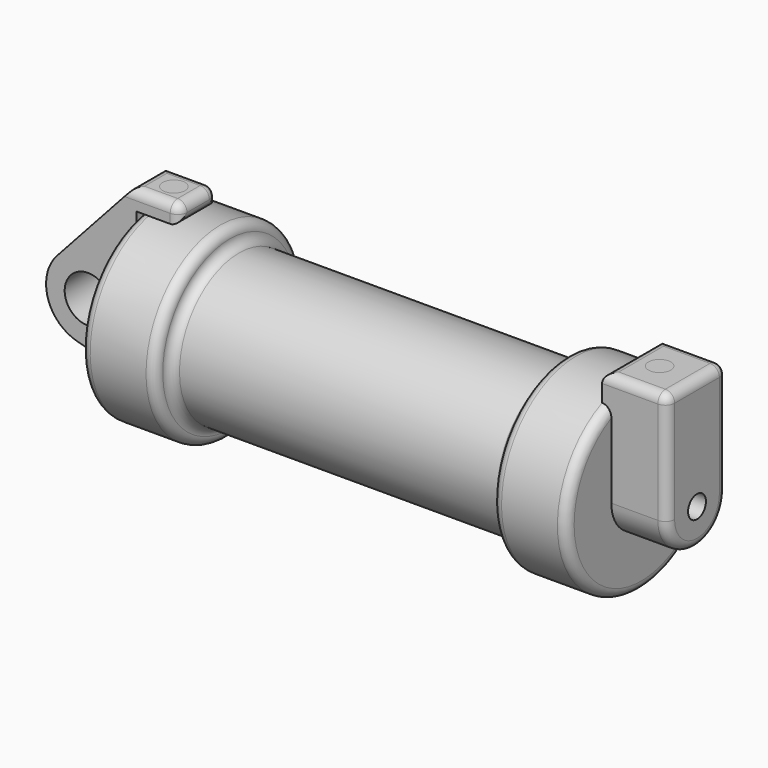
from build123d import *

# Parameters (mm, degrees)
F0_W          = 5.842
F0_H          = 12.7
F0_R          = 3.175
F2_DEPTH      = 3.175
F3_R          = 1.524
F4_DEPTH      = 7.62
F4_DEPTH_BACK = 1.27
F5_R          = 1.524
F6_DEPTH      = 17.78
F7_R          = 1.524
F8_DEPTH      = 10.414
F9_R          = 1.26999
F9_2_R        = 1.26999


# Not quite as in the source:
# - a fillet or chamfer is up to 0.001 mm smaller than in the source, because OpenCascade refuses the exact size


with BuildPart() as f1:
    # F0 (on Front) → F1 (revolve)
    with BuildSketch(Plane.XZ):
        Polygon((5.842, 12.7), (5.842, 0), (66.294, 0), (66.294, 12.7), (56.134, 12.7), (56.134, 10.16), (10.16, 10.16), (10.16, 12.7), align=None)
        with Locations((2.921, 6.35)):
            Rectangle(F0_W, F0_H)
    revolve(axis=Axis((33.147, 0, 0), (-1, 0, 0)))

    # F3 (on face) → F4 (join, two sides)
    with BuildSketch(Plane.YZ.offset(66.294)) as f4_sk:
        with BuildLine():
            ThreePointArc((-5.08, 0), (0, 5.08), (5.08, 0))
            Line((5.08, 0), (5.08, 11.6397422652))
            ThreePointArc((5.08, 11.6397422652), (0, 12.7), (-5.08, 11.6397422652))
            Line((-5.08, 11.6397422652), (-5.08, 0))
        make_face()
        with BuildLine():
            ThreePointArc((-5.08, 0), (0, -5.08), (5.08, 0))
            ThreePointArc((5.08, 0), (0, 5.08), (-5.08, 0))
        make_face()
        Circle(F3_R, mode=Mode.SUBTRACT)
        with BuildLine():
            ThreePointArc((-5.08, 11.6397422652), (0, 12.7), (5.08, 11.6397422652))
            Line((5.08, 11.6397422652), (5.08, 15.24))
            Line((5.08, 15.24), (-5.08, 15.24))
            Line((-5.08, 15.24), (-5.08, 11.6397422652))
        make_face()
    extrude(amount=F4_DEPTH)
    extrude(f4_sk.sketch, amount=-F4_DEPTH_BACK)

    # F9 (radius 1.27 in the source; OpenCascade refuses exactly that, so slightly less here)
    f9_edges = [f1.edges().sort_by_distance(p)[0] for p in [
        (10.16, 0, -12.7),
        (0, 0, -12.7),
        (10.16, 0, -10.16),
        (56.134, 0, -10.16),
        (33.147, 0, 10.16),
        (73.914, 0, 15.24),
        (69.469, 5.08, 15.24),
        (65.024, 0, 15.24),
        (69.469, -5.08, 15.24),
        (56.134, 0, -12.7),
        (66.294, 0, -12.7),
        (73.914, -5.08, 7.62),
        (73.914, 5.08, 7.62),
        (73.914, 0, -5.08),
    ]]
    fillet(f9_edges, radius=F9_R)


with BuildPart() as f2:
    # F0 (on Front) → F2 (new body, symmetric)
    with BuildSketch(Plane.XZ):
        with BuildLine():
            Line((-0.9398, 0), (0, 0))
            Line((0, 0), (0, 12.7))
            Line((0, 12.7), (5.842, 12.7))
            Line((5.842, 12.7), (5.842, 15.24))
            Line((5.842, 15.24), (-0.508, 15.24))
            Line((-0.508, 15.24), (-10.8806298187, 3.8475430269))
            ThreePointArc((-10.8806298187, 3.8475430269), (-4.5919612295, 5.3297205562), (-0.9398, 0))
        make_face()
        with BuildLine():
            ThreePointArc((-8.1826630726, -5.5069827884), (-3.1957909266, -4.5493385486), (-0.9398, 0))
            ThreePointArc((-0.9398, 0), (-4.5919612295, 5.3297205562), (-10.8806298187, 3.8475430269))
            ThreePointArc((-10.8806298187, 3.8475430269), (-12.1459778134, -1.5837270034), (-8.1826630726, -5.5069827884))
        make_face()
        with Locations((-6.6548, 0)):
            Circle(F0_R, mode=Mode.SUBTRACT)
        with BuildLine():
            Line((5.842, 0), (0, 0))
            Line((0, 0), (-0.9398, 0))
            ThreePointArc((-0.9398, 0), (-3.1957909266, -4.5493385486), (-8.1826630726, -5.5069827884))
            Line((-8.1826630726, -5.5069827884), (5.842, -9.398))
            Line((5.842, -9.398), (5.842, 0))
        make_face()
    extrude(amount=F2_DEPTH, both=True)

    # F9#2 (radius 1.27 in the source; OpenCascade refuses exactly that, so slightly less here)
    f9_2_edges = [f2.edges().sort_by_distance(p)[0] for p in [
        (5.842, 0, 15.24),
        (2.667, -3.175, 15.24),
        (5.842, 0, 12.7),
        (5.842, 3.175, 13.97),
        (5.842, -3.175, 13.97),
        (2.667, 3.175, 15.24),
        (-0.508, 0, 15.24),
    ]]
    fillet(f9_2_edges, radius=F9_2_R)


with BuildPart() as f6:
    # F5 (on face) → F6 (new body)
    with BuildSketch(Plane.XY.offset(15.24)):
        with Locations((2.5386845227, -0.0023302223)):
            Circle(F5_R)
    extrude(amount=-F6_DEPTH)


with BuildPart() as f8:
    # F7 (on face) → F8 (new body)
    with BuildSketch(Plane.XY.offset(15.24)):
        with Locations((68.828292191, -0.007390372)):
            Circle(F7_R)
    extrude(amount=-F8_DEPTH)


solid = Compound([f1.part, f2.part, f6.part, f8.part])
